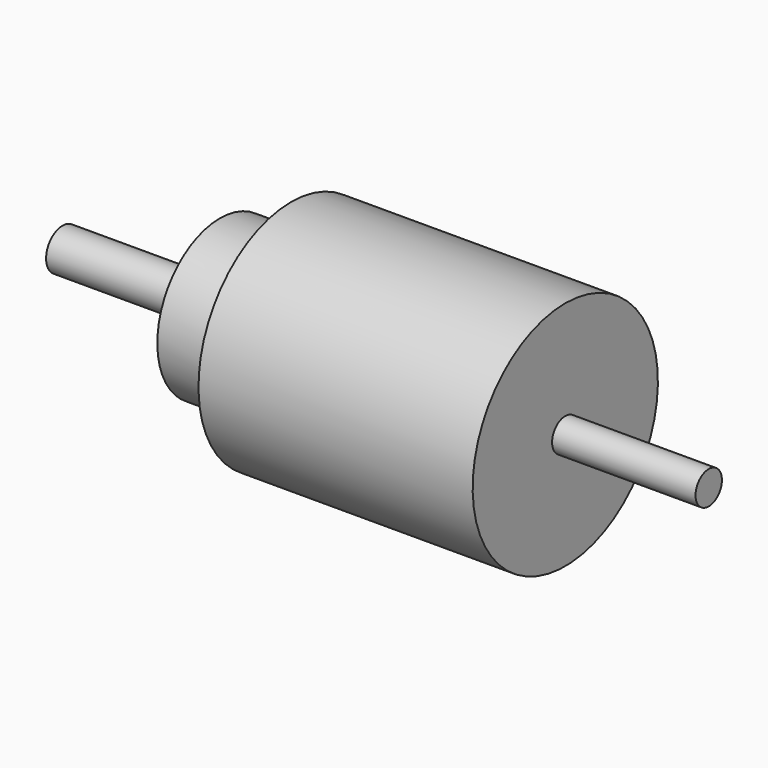
from build123d import *

# Parameters (mm, degrees)
F1_W = 17.41
F1_H = 2
F2_W = 55.31
F2_H = 2
F3_W = 19.1
F3_H = 2.5


with BuildPart() as f4:
    # F1 (on Front) → F4 (revolve)
    with BuildSketch(Plane.XZ):
        with Locations((8.705, 1)):
            Rectangle(F1_W, F1_H)
    revolve(axis=Axis((-21.8, 0, 0), (-1, 0, 0)))

    # F2 (on Front) → F5 (revolve)
    with BuildSketch(Plane.XZ):
        with Locations((-10.245, 1)):
            Rectangle(F2_W, F2_H)
    revolve(axis=Axis((-21.8, 0, 0), (-1, 0, 0)))


with BuildPart() as f4b:
    # F1 (on Front) → F4, piece 2 (revolve)
    with BuildSketch(Plane.XZ):
        Polygon((0, 14.05), (-33.2730562752, 14.05), (-35.9, 9.5), (-35.9, 2), (0, 2), align=None)
    revolve(axis=Axis((-21.8, 0, 0), (-1, 0, 0)))


with BuildPart() as f6:
    # F3 (on Front) → F6 (revolve)
    with BuildSketch(Plane.XZ):
        with Locations((-51.46, 1.25)):
            Rectangle(F3_W, F3_H)
        Polygon((-35.9, 9.5), (-41.91, 9.5), (-41.91, 2.5), (-41.91, 0), (-35.9, 0), align=None)
    revolve(axis=Axis((-21.8, 0, 0), (-1, 0, 0)))


solid = Compound([f4.part, f4b.part, f6.part])
